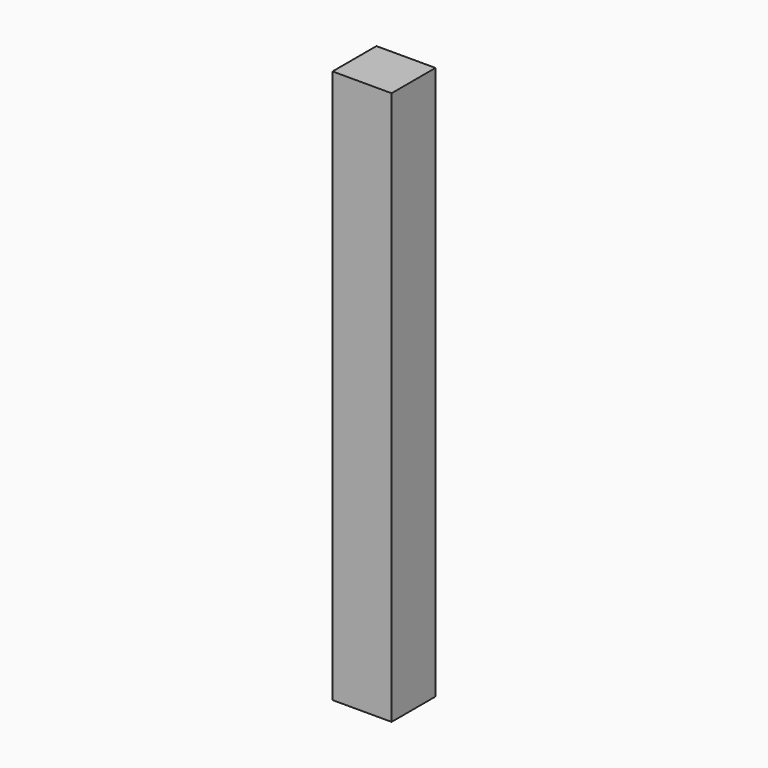
from build123d import *

# Parameters (mm, degrees)
F0_TEXT_SIZE = 33.7192271319
F1_DEPTH     = 2.54


# Not quite as in the source:
# - Text() gives the source's letters only with a copy of the font that has no kerning and outlines rounded to 1/6400 em; it was checked with that copy


with BuildPart() as f1:
    # F0 (on Front) → F1 (new body)
    with BuildSketch(Plane.XZ):
        with Locations((-7.8186457912, 0)):
            Text('l', F0_TEXT_SIZE, font='Open Sans', text_align=(TextAlign.LEFT, TextAlign.BOTTOM))
    extrude(amount=F1_DEPTH)


solid = f1.part
